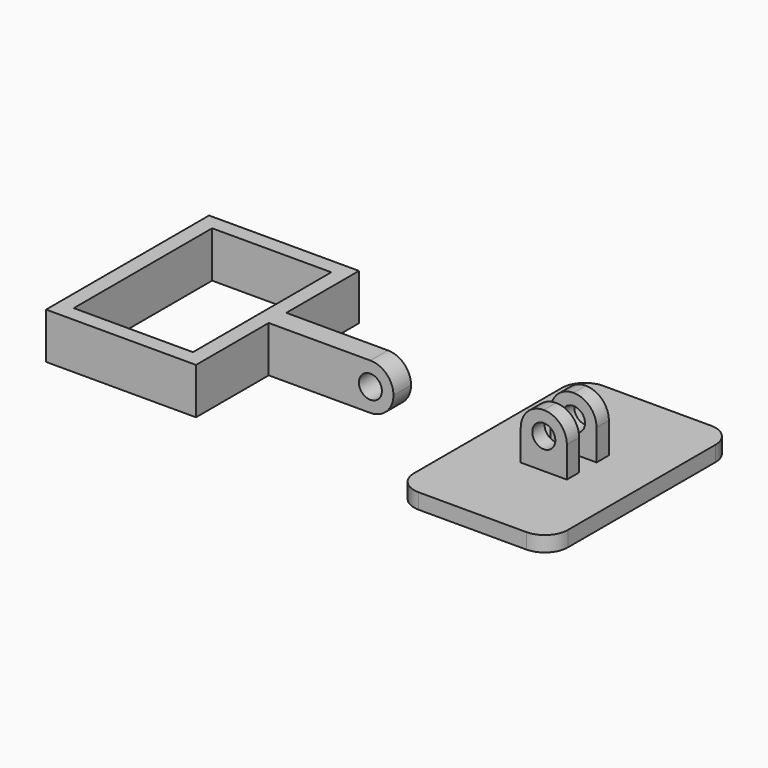
from build123d import *

# Parameters (mm, degrees)
F0_W     = 15.5
F0_H     = 22.5
F0_W_2   = 16.2271768153
F0_H_2   = 2.8558950871
F1_DEPTH = 6
F2_R     = 1.5
F3_DEPTH = 25
F4_W     = 20
F4_H     = 30
F4_W_2   = 6
F4_H_2   = 2
F5_DEPTH = 2
F6_DEPTH = 9
F7_R     = 2.99999
F7_2_R   = 2.99999
F8_R     = 1.5
F9_DEPTH = 25


# Not quite as in the source:
# - a fillet or chamfer is up to 0.001 mm smaller than in the source, because OpenCascade refuses the exact size


with BuildPart() as f1:
    # F0 (on Top) → F1 (new body)
    with BuildSketch(Plane.XY):
        Polygon((-9.75, -13.25), (9.75, -13.25), (9.75, -1.4279475436), (9.75, 1.4279475436), (9.75, 13.25), (-9.75, 13.25), align=None)
        Rectangle(F0_W, F0_H, mode=Mode.SUBTRACT)
        with Locations((17.8635884076, 0)):
            Rectangle(F0_W_2, F0_H_2)
    extrude(amount=F1_DEPTH)

    # F2 (on face) → F3 (cut)
    with BuildSketch(Plane.XZ.offset(1.4279475436)):
        with Locations((22.9771768153, 3)):
            Circle(F2_R)
    extrude(amount=-F3_DEPTH, mode=Mode.SUBTRACT)

    # F7 (radius 3 in the source; OpenCascade refuses exactly that, so slightly less here)
    f7_edges = [f1.edges().sort_by_distance(p)[0] for p in [
        (25.977177, 0, 0),
        (25.977177, 0, 6),
    ]]
    fillet(f7_edges, radius=F7_R)


with BuildPart() as f5:
    # F4 (on Top) → F5 (new body)
    with BuildSketch(Plane.XY):
        with Locations((47.1228286624, 0)):
            Rectangle(F4_W, F4_H)
        with Locations((47.1228286624, -2.4156674554)):
            Rectangle(F4_W_2, F4_H_2, mode=Mode.SUBTRACT)
        with Locations((47.1228286624, 2.4156674554)):
            Rectangle(F4_W_2, F4_H_2, mode=Mode.SUBTRACT)
        with Locations((47.1228286624, 2.4156674554)):
            Rectangle(F4_W_2, F4_H_2)
        with Locations((47.1228286624, -2.4156674554)):
            Rectangle(F4_W_2, F4_H_2)
    extrude(amount=F5_DEPTH)

    # F4 (on Top) → F6 (join)
    with BuildSketch(Plane.XY):
        with Locations((47.1228286624, 2.4156674554)):
            Rectangle(F4_W_2, F4_H_2)
        with Locations((47.1228286624, -2.4156674554)):
            Rectangle(F4_W_2, F4_H_2)
    extrude(amount=F6_DEPTH)

    # F7#2 (radius 3 in the source; OpenCascade refuses exactly that, so slightly less here)
    f7_2_edges = [f5.edges().sort_by_distance(p)[0] for p in [
        (44.122829, 2.415667, 9),
        (44.122829, -2.415667, 9),
        (50.122829, 2.415667, 9),
        (50.122829, -2.415667, 9),
        (37.122829, -15, 1),
        (57.122829, -15, 1),
        (57.122829, 15, 1),
        (37.122829, 15, 1),
    ]]
    fillet(f7_2_edges, radius=F7_2_R)

    # F8 (on face) → F9 (cut)
    with BuildSketch(Plane.XZ.offset(3.4156674554)):
        with Locations((47.1228286624, 6)):
            Circle(F8_R)
    extrude(amount=-F9_DEPTH, mode=Mode.SUBTRACT)


solid = Compound([f1.part, f5.part])
